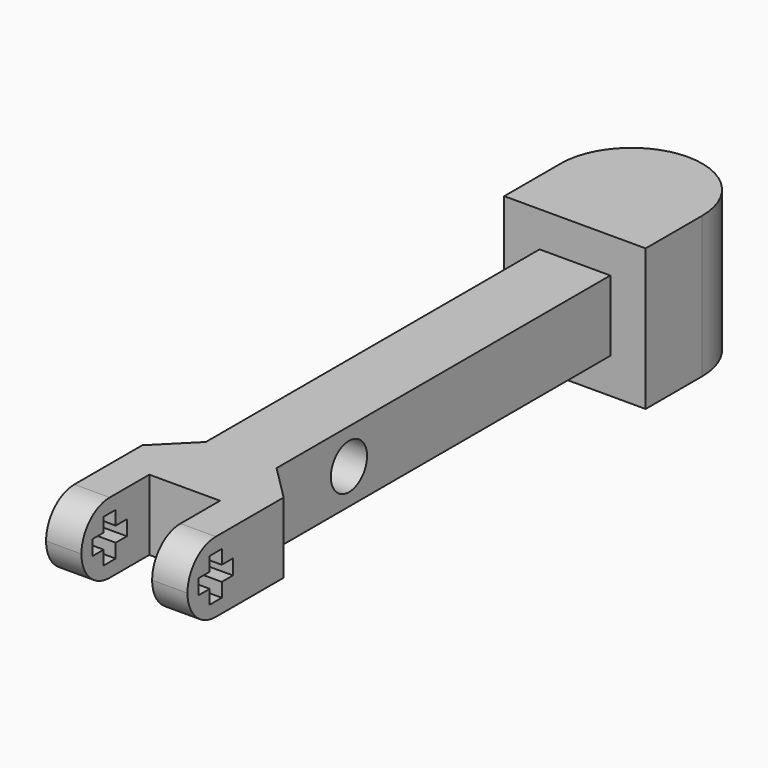
from build123d import *

# Parameters (mm, degrees)
F1_DEPTH = 7.9375
F2_R     = 2.54
F2_W     = 1.6891
F2_H     = 1.56845
F2_H_2   = 1.6891
F2_W_2   = 1.56845
F3_DEPTH = 15.875
F4_SIZE  = 3.96874
F5_W     = 15.875
F5_H     = 15.875
F6_DEPTH = 15.875
F7_R     = 7.93749


# Not quite as in the source:
# - a fillet or chamfer is up to 0.001 mm smaller than in the source, because OpenCascade refuses the exact size


with BuildPart() as f1:
    # F0 (on Top) → F1 (new body)
    with BuildSketch(Plane.XY):
        Polygon((3.96875, 0), (0, 0), (0, -13.49375), (3.96875, -13.49375), (3.96875, -3.96875), (11.90625, -3.96875), (11.90625, -13.49375), (15.875, -13.49375), (15.875, 0), (11.90625, 0), (11.90625, 50.8), (3.96875, 50.8), align=None)
    extrude(amount=F1_DEPTH)

    # F2 (on face) → F3 (cut, through all)
    with BuildSketch(Plane.YZ.offset(15.875)):
        with BuildLine():
            ThreePointArc((-9.525, 0), (-12.3313300378, 1.1624199622), (-13.49375, 3.96875))
            Line((-13.49375, 3.96875), (-13.49375, 0))
            Line((-13.49375, 0), (-9.525, 0))
        make_face()
        with BuildLine():
            ThreePointArc((-13.49375, 3.96875), (-12.3313300378, 6.7750800378), (-9.525, 7.9375))
            Line((-9.525, 7.9375), (-13.49375, 7.9375))
            Line((-13.49375, 7.9375), (-13.49375, 3.96875))
        make_face()
        with Locations((14.128559196, 3.96875)):
            Circle(F2_R)
        with Locations((-9.525, 5.597525)):
            Rectangle(F2_W, F2_H)
        with Locations((-9.525, 3.96875)):
            Rectangle(F2_W, F2_H_2)
        with Locations((-11.153775, 3.96875)):
            Rectangle(F2_W_2, F2_H_2)
        with Locations((-7.896225, 3.96875)):
            Rectangle(F2_W_2, F2_H_2)
        with Locations((-9.525, 2.339975)):
            Rectangle(F2_W, F2_H)
    extrude(amount=-F3_DEPTH, mode=Mode.SUBTRACT)

    # F4 (size 3.96875 in the source; OpenCascade refuses exactly that, so slightly less here)
    f4_edges = [f1.edges().sort_by_distance(p)[0] for p in [
        (11.90625, 0, 3.96875),
        (3.96875, 0, 3.96875),
    ]]
    chamfer(f4_edges, length=F4_SIZE)

    # F5 (on face) → F6 (join)
    with BuildSketch(Plane(origin=(0, 50.8, 0), x_dir=(-1, 0, 0), z_dir=(0, 1, 0))):
        with Locations((-7.9375, 3.96875)):
            Rectangle(F5_W, F5_H)
    extrude(amount=F6_DEPTH)

    # F7 (radius 7.9375 in the source; OpenCascade refuses exactly that, so slightly less here)
    f7_edges = [f1.edges().sort_by_distance(p)[0] for p in [
        (15.875, 66.675, 3.96875),
        (0, 66.675, 3.96875),
    ]]
    fillet(f7_edges, radius=F7_R)


solid = f1.part
